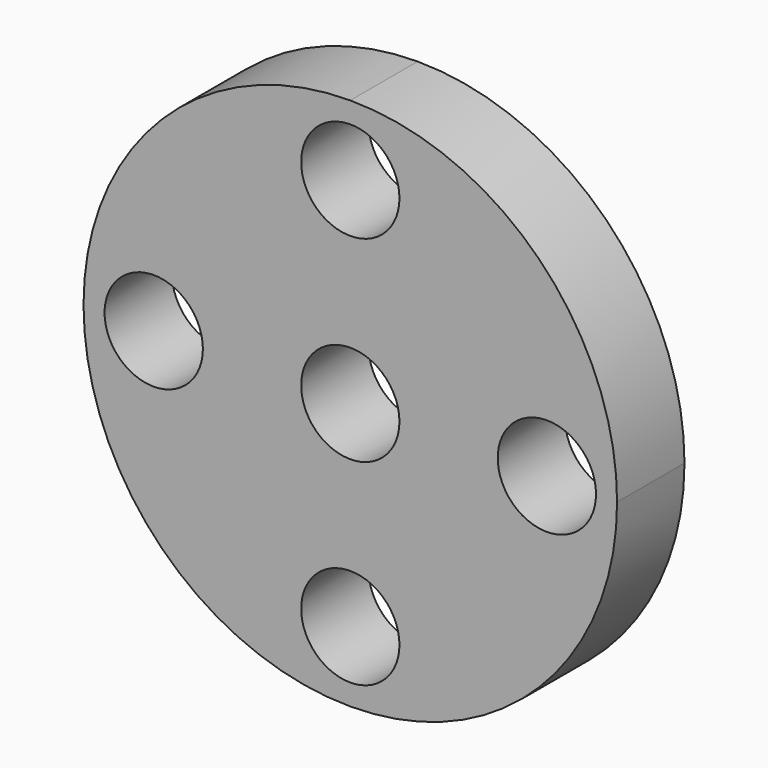
from build123d import *

# Parameters (mm, degrees)
F0_R     = 4.445
F1_DEPTH = 7.62


# Not quite as in the source:
# - a feature names something its author has since deleted; it is built from what else it names


with BuildPart() as f1:
    # F0 (on Front) → F1 (new body)
    with BuildSketch(Plane.XZ):
        with BuildLine():
            Line((6.35, 17.78), (6.35, 6.35))
            Line((6.35, 6.35), (17.78, 6.35))
            ThreePointArc((17.78, 6.35), (22.2701280605, 4.4901280605), (24.13, 0))
            ThreePointArc((24.13, 0), (17.06248663, 17.06248663), (0, 24.13))
            ThreePointArc((0, 24.13), (4.4901280605, 22.2701280605), (6.35, 17.78))
        make_face()
        with BuildLine():
            Line((17.78, -6.35), (6.35, -6.35))
            Line((6.35, -6.35), (6.35, -17.78))
            ThreePointArc((6.35, -17.78), (4.4901280329, -22.2701280882), (-7.83e-08, -24.13))
            ThreePointArc((-7.83e-08, -24.13), (17.0624866024, -17.0624866577), (24.13, 0))
            ThreePointArc((24.13, 0), (22.2701280605, -4.4901280605), (17.78, -6.35))
        make_face()
        with BuildLine():
            Line((-17.78, 6.35), (-6.35, 6.35))
            Line((-6.35, 6.35), (-6.35, 17.78))
            ThreePointArc((-6.35, 17.78), (-4.4901280605, 22.2701280605), (0, 24.13))
            ThreePointArc((0, 24.13), (-17.0624866246, 17.0624866355), (-24.13, 1.54e-08))
            ThreePointArc((-24.13, 1.54e-08), (-22.2701280551, 4.490128066), (-17.78, 6.35))
        make_face()
        with BuildLine():
            Line((-6.35, -17.78), (-6.35, -6.35))
            Line((-6.35, -6.35), (-17.78, -6.35))
            ThreePointArc((-17.78, -6.35), (-22.270128066, -4.4901280551), (-24.13, 1.54e-08))
            ThreePointArc((-24.13, 1.54e-08), (-17.0624866631, -17.0624865969), (-7.83e-08, -24.13))
            ThreePointArc((-7.83e-08, -24.13), (-4.4901280882, -22.2701280329), (-6.35, -17.78))
        make_face()
        with BuildLine():
            ThreePointArc((-6.35, 17.78), (0, 11.43), (6.35, 17.78))
            ThreePointArc((6.35, 17.78), (4.4901280605, 22.2701280605), (0, 24.13))
            ThreePointArc((0, 24.13), (-4.4901280605, 22.2701280605), (-6.35, 17.78))
        make_face()
        with Locations((0, 17.78)):
            Circle(F0_R, mode=Mode.SUBTRACT)
        with BuildLine():
            ThreePointArc((24.13, 0), (22.2701280605, 4.4901280605), (17.78, 6.35))
            ThreePointArc((17.78, 6.35), (11.43, 0), (17.78, -6.35))
            ThreePointArc((17.78, -6.35), (22.2701280605, -4.4901280605), (24.13, 0))
        make_face()
        with Locations((17.78, 0)):
            Circle(F0_R, mode=Mode.SUBTRACT)
        with BuildLine():
            ThreePointArc((-7.83e-08, -24.13), (4.4901280329, -22.2701280882), (6.35, -17.78))
            ThreePointArc((6.35, -17.78), (0, -11.43), (-6.35, -17.78))
            ThreePointArc((-6.35, -17.78), (-4.4901280882, -22.2701280329), (-7.83e-08, -24.13))
        make_face()
        with Locations((0, -17.78)):
            Circle(F0_R, mode=Mode.SUBTRACT)
        with BuildLine():
            ThreePointArc((-11.43, 0), (-13.2898719395, 4.4901280605), (-17.78, 6.35))
            ThreePointArc((-17.78, 6.35), (-22.2701280551, 4.490128066), (-24.13, 1.54e-08))
            ThreePointArc((-24.13, 1.54e-08), (-22.270128066, -4.4901280551), (-17.78, -6.35))
            ThreePointArc((-17.78, -6.35), (-13.2898719395, -4.4901280605), (-11.43, 0))
        make_face()
        with Locations((-17.78, 0)):
            Circle(F0_R, mode=Mode.SUBTRACT)
        with BuildLine():
            ThreePointArc((0, -6.35), (4.4901280605, -4.4901280605), (6.35, 0))
            ThreePointArc((6.35, 0), (4.4901280605, 4.4901280605), (0, 6.35))
            ThreePointArc((0, 6.35), (-4.4901280605, 4.4901280605), (-6.35, 0))
            ThreePointArc((-6.35, 0), (-4.4901280605, -4.4901280605), (0, -6.35))
        make_face()
        Circle(F0_R, mode=Mode.SUBTRACT)
        with BuildLine():
            ThreePointArc((-6.35, 0), (-4.4901280605, 4.4901280605), (0, 6.35))
            Line((0, 6.35), (-6.35, 6.35))
            Line((-6.35, 6.35), (-6.35, 0))
        make_face()
        with BuildLine():
            Line((-6.35, -6.35), (0, -6.35))
            ThreePointArc((0, -6.35), (-4.4901280605, -4.4901280605), (-6.35, 0))
            Line((-6.35, 0), (-6.35, -6.35))
        make_face()
        with BuildLine():
            Line((6.35, -6.35), (6.35, 0))
            ThreePointArc((6.35, 0), (4.4901280605, -4.4901280605), (0, -6.35))
            Line((0, -6.35), (6.35, -6.35))
        make_face()
        with BuildLine():
            ThreePointArc((0, 6.35), (4.4901280605, 4.4901280605), (6.35, 0))
            Line((6.35, 0), (6.35, 6.35))
            Line((6.35, 6.35), (0, 6.35))
        make_face()
        with BuildLine():
            Line((-6.35, -6.35), (-6.35, 0))
            Line((-6.35, 0), (-6.35, 6.35))
            Line((-6.35, 6.35), (-17.78, 6.35))
            ThreePointArc((-17.78, 6.35), (-13.2898719395, 4.4901280605), (-11.43, 0))
            ThreePointArc((-11.43, 0), (-13.2898719395, -4.4901280605), (-17.78, -6.35))
            Line((-17.78, -6.35), (-6.35, -6.35))
        make_face()
        with BuildLine():
            Line((6.35, -6.35), (0, -6.35))
            Line((0, -6.35), (-6.35, -6.35))
            Line((-6.35, -6.35), (-6.35, -17.78))
            ThreePointArc((-6.35, -17.78), (0, -11.43), (6.35, -17.78))
            Line((6.35, -17.78), (6.35, -6.35))
        make_face()
        with BuildLine():
            Line((6.35, 6.35), (6.35, 0))
            Line((6.35, 0), (6.35, -6.35))
            Line((6.35, -6.35), (17.78, -6.35))
            ThreePointArc((17.78, -6.35), (11.43, 0), (17.78, 6.35))
            Line((17.78, 6.35), (6.35, 6.35))
        make_face()
        with BuildLine():
            Line((-6.35, 6.35), (0, 6.35))
            Line((0, 6.35), (6.35, 6.35))
            Line((6.35, 6.35), (6.35, 17.78))
            ThreePointArc((6.35, 17.78), (0, 11.43), (-6.35, 17.78))
            Line((-6.35, 17.78), (-6.35, 6.35))
        make_face()
    extrude(amount=F1_DEPTH)


solid = f1.part
